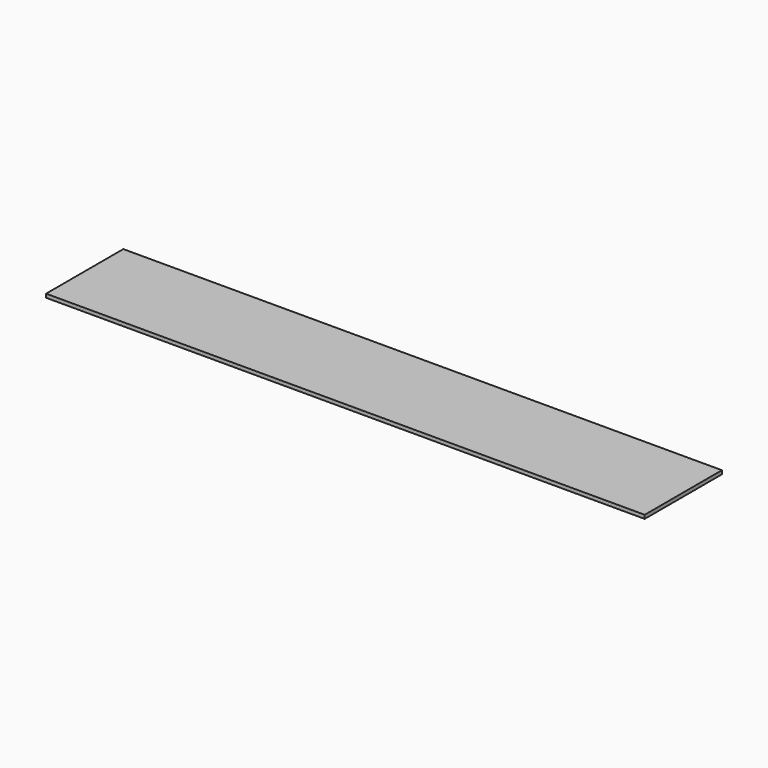
from build123d import *

# Parameters (mm, degrees)
F0_W     = 521
F0_H     = 84
F1_DEPTH = 3.175


# Not quite as in the source:
# - a length typed as a fraction of an inch, garbled in the dataset ("3 / 203.2 mm" for 3/8 in), is restored


with BuildPart() as f1:
    # F0 (on Top) → F1 (new body)
    with BuildSketch(Plane.XY):
        Rectangle(F0_W, F0_H)
    extrude(amount=F1_DEPTH)


solid = f1.part
